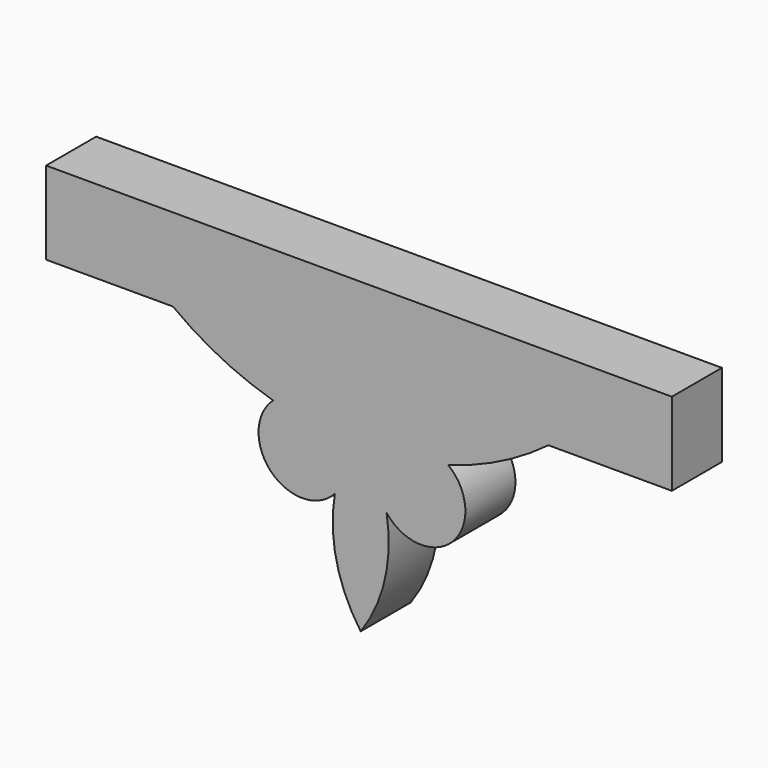
from build123d import *

# Parameters (mm, degrees)
F1_DEPTH = 5


# Not quite as in the source:
# - a feature of the source that left no trace in its solid (it failed there, or was rolled back) is left out


with BuildPart() as f1:
    # F0 (on Front) → F1 (new body)
    with BuildSketch(Plane.XZ):
        Polygon((32.530919835, 39.797769749), (-17.469080165, 39.797769749), (-17.469080165, 33.1753157079), (-7.3289242573, 33.1753157079), (22.6710757427, 33.1753157079), (32.530919835, 33.1753157079), align=None)
        with BuildLine():
            Line((22.6710757427, 33.1753157079), (-7.3289242573, 33.1753157079))
            ThreePointArc((-7.3289242573, 33.1753157079), (-3.5071800034, 30.8135939836), (0.6755496306, 29.1740112764))
            Line((0.6755496306, 29.1740112764), (7.6710757427, 29.1740112764))
            Line((7.6710757427, 29.1740112764), (14.6666018548, 29.1740112764))
            ThreePointArc((14.6666018548, 29.1740112764), (18.8493314888, 30.8135939836), (22.6710757427, 33.1753157079))
        make_face()
        with BuildLine():
            Line((7.6710757427, 29.1740112764), (0.6755496306, 29.1740112764))
            ThreePointArc((0.6755496306, 29.1740112764), (0.5215760436, 24.0947560366), (5.6017371537, 24.215191712))
            ThreePointArc((5.6017371537, 24.215191712), (6.355285365, 26.8119146366), (7.6710757427, 29.1740112764))
        make_face()
        with BuildLine():
            ThreePointArc((9.7404143316, 24.215191712), (15.0089010531, 23.907669722), (14.6666018548, 29.1740112764))
            Line((14.6666018548, 29.1740112764), (7.6710757427, 29.1740112764))
            ThreePointArc((7.6710757427, 29.1740112764), (8.9868661204, 26.8119146366), (9.7404143316, 24.215191712))
        make_face()
        with BuildLine():
            ThreePointArc((9.7404143316, 24.215191712), (8.9868661204, 26.8119146366), (7.6710757427, 29.1740112764))
            ThreePointArc((7.6710757427, 29.1740112764), (6.355285365, 26.8119146366), (5.6017371537, 24.215191712))
            ThreePointArc((5.6017371537, 24.215191712), (5.7343151874, 19.5038742549), (7.6710757427, 15.20700939))
            ThreePointArc((7.6710757427, 15.20700939), (9.607836298, 19.5038742549), (9.7404143316, 24.215191712))
        make_face()
    extrude(amount=F1_DEPTH)


solid = f1.part
